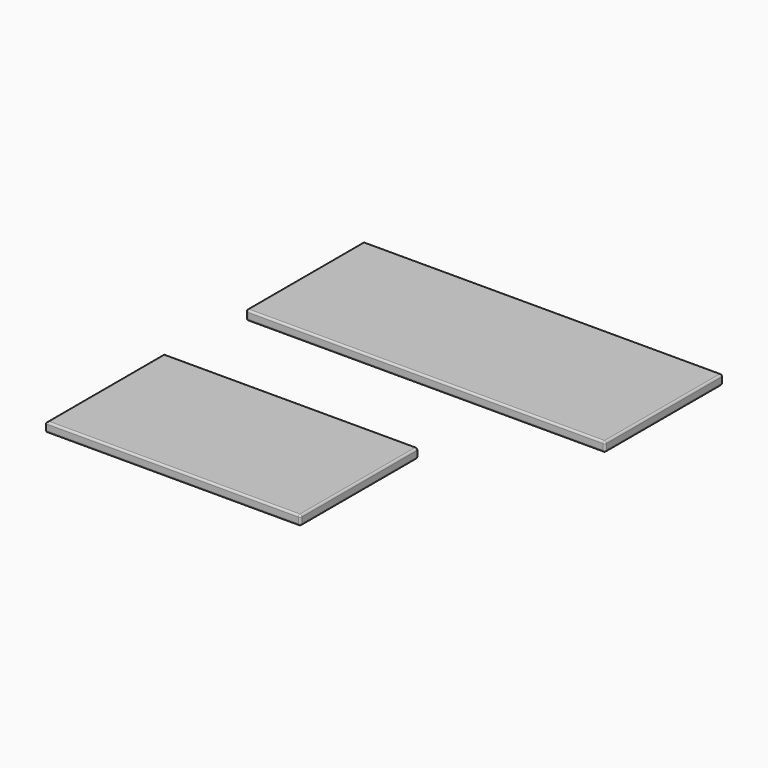
from build123d import *

# Parameters (mm, degrees)
F0_W     = 655
F0_H     = 380
F1_DEPTH = 25
F3_DEPTH = 380.001
F4_R     = 5
F5_W     = 925
F5_H     = 380
F6_DEPTH = 25
F7_R     = 5


with BuildPart() as f1:
    # F0 (on Top) → F1 (new body)
    with BuildSketch(Plane.XY):
        with Locations((46.5359067917, -670.1017089717)):
            Rectangle(F0_W, F0_H)
    extrude(amount=F1_DEPTH)

    # F2 (on face) → F3 (cut, through all)
    with BuildSketch(Plane.XZ.offset(860.1017089717)):
        Polygon((-329.5351266861, 5.0213485956), (-321.2029933929, 5.0213038921), (-293.8260436058, 27.9015563428), (-329.5351266861, 27.9015563428), align=None)
    extrude(amount=-F3_DEPTH, mode=Mode.SUBTRACT)

    # F4
    f4_edges = [f1.edges().sort_by_distance(p)[0] for p in [
        (-280.964093, -670.101709, 25),
        (46.535907, -860.101709, 25),
        (374.035907, -670.101709, 25),
        (46.535907, -480.101709, 25),
        (-280.964093, -670.101709, 0),
        (46.535907, -860.101709, 0),
        (374.035907, -670.101709, 0),
        (46.535907, -480.101709, 0),
        (374.035907, -860.101709, 12.5),
        (374.035907, -480.101709, 12.5),
    ]]
    fillet(f4_edges, radius=F4_R)


with BuildPart() as f6:
    # F5 (on Top) → F6 (new body)
    with BuildSketch(Plane.XY):
        with Locations((189.8969432941, -37.2657254338)):
            Rectangle(F5_W, F5_H)
    extrude(amount=F6_DEPTH)

    # F7
    f7_edges = [f6.edges().sort_by_distance(p)[0] for p in [
        (652.396943, -37.265725, 25),
        (189.896943, 152.734275, 25),
        (-272.603057, -37.265725, 25),
        (189.896943, -227.265725, 25),
        (652.396943, -37.265725, 0),
        (189.896943, 152.734275, 0),
        (-272.603057, -37.265725, 0),
        (189.896943, -227.265725, 0),
        (652.396943, 152.734275, 12.5),
        (-272.603057, 152.734275, 12.5),
        (-272.603057, -227.265725, 12.5),
        (652.396943, -227.265725, 12.5),
    ]]
    fillet(f7_edges, radius=F7_R)


solid = Compound([f1.part, f6.part])
